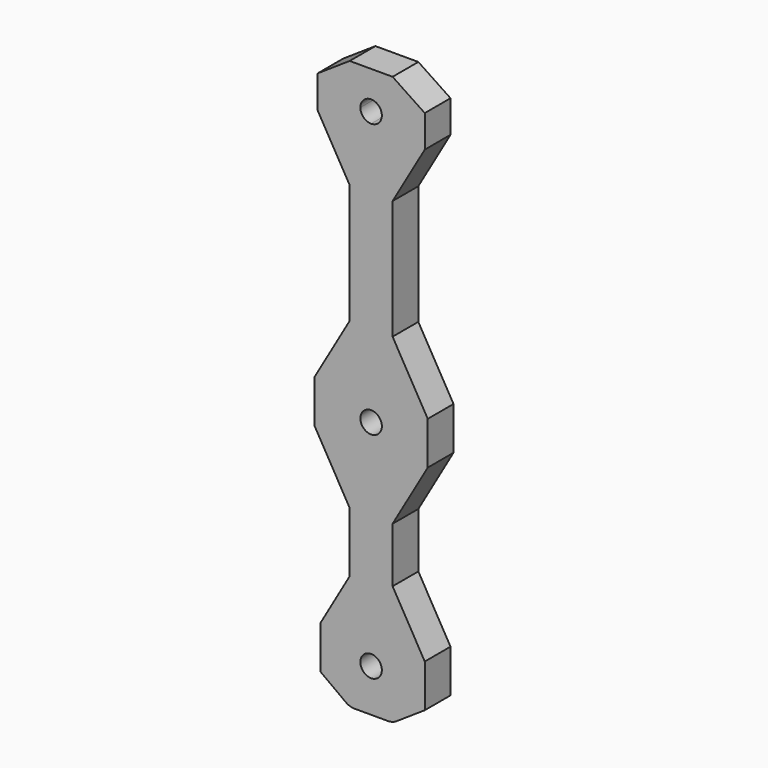
from build123d import *

# Parameters (mm, degrees)
F0_W     = 17.2899770278
F0_H     = 12.7
F0_W_2   = 19.05
F0_W_3   = 20.8100229722
F0_H_2   = 9.525
F1_DEPTH = 19.05
F2_R     = 8.89


# Not quite as in the source:
# - a feature names something its author has since deleted; it is built from what else it names


with BuildPart() as f1:
    # F0 (on Front) → F1 (new body)
    with BuildSketch(Plane.XZ):
        with BuildLine():
            Line((-48.4576454937, -259.1044321158), (-48.4576454937, -271.8044321158))
            Line((-48.4576454937, -271.8044321158), (-23.0576454937, -271.8044321158))
            Line((-23.0576454937, -271.8044321158), (-23.0576454937, -259.1044321158))
            Line((-23.0576454937, -259.1044321158), (-23.0576454937, -246.4044321158))
            Line((-23.0576454937, -246.4044321158), (-29.4076454937, -246.4044321158))
            ThreePointArc((-29.4076454937, -246.4044321158), (-35.7576454937, -252.7544321158), (-42.1076454937, -246.4044321158))
            Line((-42.1076454937, -246.4044321158), (-48.4576454937, -246.4044321158))
            Line((-48.4576454937, -246.4044321158), (-48.4576454937, -259.1044321158))
        make_face()
        Polygon((-65.7476225216, -259.1044321158), (-48.4576454937, -271.8044321158), (-48.4576454937, -259.1044321158), align=None)
        Polygon((-23.0576454937, -259.1044321158), (-23.0576454937, -271.8044321158), (-4.0076454937, -259.1044321158), align=None)
        with Locations((-57.1026340077, -252.7544321158)):
            Rectangle(F0_W, F0_H)
        with Locations((-13.5326454937, -252.7544321158)):
            Rectangle(F0_W_2, F0_H)
        with Locations((-57.1026340077, -240.0544321158)):
            Rectangle(F0_W, F0_H)
        with BuildLine():
            Line((-48.4576454937, -233.7044321158), (-48.4576454937, -246.4044321158))
            Line((-48.4576454937, -246.4044321158), (-42.1076454937, -246.4044321158))
            ThreePointArc((-42.1076454937, -246.4044321158), (-35.7576454937, -240.0544321158), (-29.4076454937, -246.4044321158))
            Line((-29.4076454937, -246.4044321158), (-23.0576454937, -246.4044321158))
            Line((-23.0576454937, -246.4044321158), (-23.0576454937, -233.7044321158))
            Line((-23.0576454937, -233.7044321158), (-23.0576454937, -200.7088642316))
            Line((-23.0576454937, -200.7088642316), (-23.0576454937, -168.1484492103))
            Line((-23.0576454937, -168.1484492103), (-23.0576454937, -132.1044321158))
            Line((-23.0576454937, -132.1044321158), (-23.0576454937, -119.4044321158))
            Line((-23.0576454937, -119.4044321158), (-29.4076454937, -119.4044321158))
            ThreePointArc((-29.4076454937, -119.4044321158), (-35.7576454937, -125.7544321158), (-42.1076454937, -119.4044321158))
            Line((-42.1076454937, -119.4044321158), (-48.4576454937, -119.4044321158))
            Line((-48.4576454937, -119.4044321158), (-48.4576454937, -132.1044321158))
            Line((-48.4576454937, -132.1044321158), (-48.4576454937, -168.1484492103))
            Line((-48.4576454937, -168.1484492103), (-48.4576454937, -203.7573134419))
            Line((-48.4576454937, -203.7573134419), (-48.4576454937, -233.7044321158))
        make_face()
        with Locations((-13.5326454937, -240.0544321158)):
            Rectangle(F0_W_2, F0_H)
        Polygon((-65.7476225216, -233.7044321158), (-48.4576454937, -233.7044321158), (-48.4576454937, -203.7573134419), align=None)
        Polygon((-23.0576454937, -200.7088642316), (-23.0576454937, -233.7044321158), (-4.0076454937, -233.7044321158), align=None)
        Polygon((-69.2676684659, -132.1044321158), (-48.4576454937, -168.1484492103), (-48.4576454937, -132.1044321158), align=None)
        Polygon((-23.0576454937, -132.1044321158), (-23.0576454937, -168.1484492103), (-2.2476225216, -132.1044321158), align=None)
        with Locations((-58.8626569798, -125.7544321158)):
            Rectangle(F0_W_3, F0_H)
        with Locations((-12.6526340077, -125.7544321158)):
            Rectangle(F0_W_3, F0_H)
        with Locations((-58.8626569798, -113.0544321158)):
            Rectangle(F0_W_3, F0_H)
        with BuildLine():
            Line((-48.4576454937, -106.7044321158), (-48.4576454937, -119.4044321158))
            Line((-48.4576454937, -119.4044321158), (-42.1076454937, -119.4044321158))
            ThreePointArc((-42.1076454937, -119.4044321158), (-35.7576454937, -113.0544321158), (-29.4076454937, -119.4044321158))
            Line((-29.4076454937, -119.4044321158), (-23.0576454937, -119.4044321158))
            Line((-23.0576454937, -119.4044321158), (-23.0576454937, -106.7044321158))
            Line((-23.0576454937, -106.7044321158), (-23.0576454937, -70.6604150213))
            Line((-23.0576454937, -70.6604150213), (-23.0576454937, 0))
            Line((-23.0576454937, 0), (-23.0576454937, 32.9955678842))
            Line((-23.0576454937, 32.9955678842), (-35.7576454937, 32.9955678842))
            Line((-35.7576454937, 32.9955678842), (-48.4576454937, 32.9955678842))
            Line((-48.4576454937, 32.9955678842), (-48.4576454937, 0))
            Line((-48.4576454937, 0), (-48.4576454937, -70.6604150213))
            Line((-48.4576454937, -70.6604150213), (-48.4576454937, -106.7044321158))
        make_face()
        with Locations((-12.6526340077, -113.0544321158)):
            Rectangle(F0_W_3, F0_H)
        Polygon((-69.2676684659, -106.7044321158), (-48.4576454937, -106.7044321158), (-48.4576454937, -70.6604150213), align=None)
        Polygon((-23.0576454937, -70.6604150213), (-23.0576454937, -106.7044321158), (-2.2476225216, -106.7044321158), align=None)
        Polygon((-67.5076454937, 32.9955678842), (-48.4576454937, 0), (-48.4576454937, 32.9955678842), align=None)
        Polygon((-23.0576454937, 32.9955678842), (-23.0576454937, 0), (-4.0076454937, 32.9955678842), align=None)
        with Locations((-57.9826454937, 37.7580678842)):
            Rectangle(F0_W_2, F0_H_2)
        with Locations((-13.5326454937, 37.7580678842)):
            Rectangle(F0_W_2, F0_H_2)
        with Locations((-57.9826454937, 47.2830678842)):
            Rectangle(F0_W_2, F0_H_2)
        with Locations((-13.5326454937, 47.2830678842)):
            Rectangle(F0_W_2, F0_H_2)
        Polygon((-48.4576454937, 64.7455678842), (-48.4576454937, 52.0455678842), (-35.7576454937, 52.0455678842), (-23.0576454937, 52.0455678842), (-23.0576454937, 64.7455678842), align=None)
        Polygon((-67.5076454937, 52.0455678842), (-48.4576454937, 52.0455678842), (-48.4576454937, 64.7455678842), align=None)
        Polygon((-23.0576454937, 64.7455678842), (-23.0576454937, 52.0455678842), (-4.0076454937, 52.0455678842), align=None)
        with BuildLine():
            Line((-29.4076454937, 42.5205678842), (-23.0576454937, 42.5205678842))
            Line((-23.0576454937, 42.5205678842), (-23.0576454937, 52.0455678842))
            Line((-23.0576454937, 52.0455678842), (-35.7576454937, 52.0455678842))
            Line((-35.7576454937, 52.0455678842), (-35.7576454937, 48.8705678842))
            ThreePointArc((-35.7576454937, 48.8705678842), (-31.2675174332, 47.0106959447), (-29.4076454937, 42.5205678842))
        make_face()
        with BuildLine():
            Line((-48.4576454937, 52.0455678842), (-48.4576454937, 42.5205678842))
            Line((-48.4576454937, 42.5205678842), (-42.1076454937, 42.5205678842))
            ThreePointArc((-42.1076454937, 42.5205678842), (-40.2477735543, 47.0106959447), (-35.7576454937, 48.8705678842))
            Line((-35.7576454937, 48.8705678842), (-35.7576454937, 52.0455678842))
            Line((-35.7576454937, 52.0455678842), (-48.4576454937, 52.0455678842))
        make_face()
        with BuildLine():
            Line((-35.7576454937, 32.9955678842), (-23.0576454937, 32.9955678842))
            Line((-23.0576454937, 32.9955678842), (-23.0576454937, 42.5205678842))
            Line((-23.0576454937, 42.5205678842), (-29.4076454937, 42.5205678842))
            ThreePointArc((-29.4076454937, 42.5205678842), (-31.2675174332, 38.0304398237), (-35.7576454937, 36.1705678842))
            Line((-35.7576454937, 36.1705678842), (-35.7576454937, 32.9955678842))
        make_face()
        with BuildLine():
            Line((-48.4576454937, 42.5205678842), (-48.4576454937, 32.9955678842))
            Line((-48.4576454937, 32.9955678842), (-35.7576454937, 32.9955678842))
            Line((-35.7576454937, 32.9955678842), (-35.7576454937, 36.1705678842))
            ThreePointArc((-35.7576454937, 36.1705678842), (-40.2477735543, 38.0304398237), (-42.1076454937, 42.5205678842))
            Line((-42.1076454937, 42.5205678842), (-48.4576454937, 42.5205678842))
        make_face()
    extrude(amount=F1_DEPTH)

    # F2
    f2_edges = [f1.edges().sort_by_distance(p)[0] for p in [
        (-23.057645, -9.525, -271.804432),
        (-48.457645, -9.525, -271.804432),
    ]]
    fillet(f2_edges, radius=F2_R)


solid = f1.part
